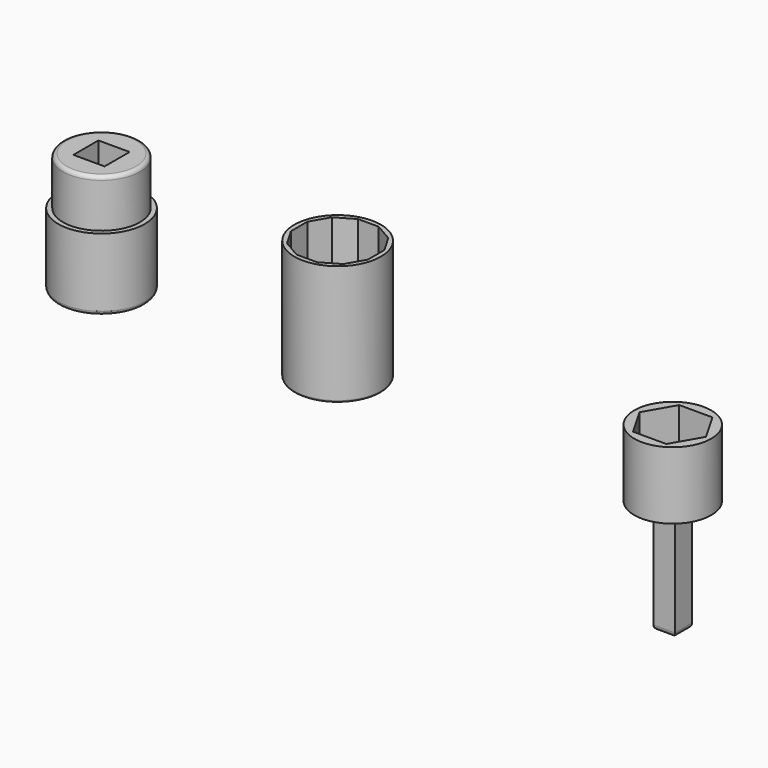
from build123d import *

# Parameters (mm, degrees)
F0_R      = 9
F0_W      = 10
F0_H      = 10
F1_DEPTH  = 12.5
F2_R      = 0.4
F3_R      = 9
F4_DEPTH  = 12.5
F6_DEPTH  = 10
F7_R      = 8
F8_DEPTH  = 14
F10_DEPTH = 23.5
F11_R     = 3.5
F12_DEPTH = 12
F13_R     = 1
F14_R     = 9
F15_DEPTH = 15
F16_R     = 8
F17_DEPTH = 10
F19_DEPTH = 14
F20_W     = 6.5
F20_H     = 6.5
F21_DEPTH = 25
F24_DEPTH = 10


# Not quite as in the source:
# - a fillet or chamfer that OpenCascade refuses, or shapes differently, is made with other operations: its cross-section is extruded or revolved along the edge and cut away or added
# - a feature names something its author has since deleted; it is built from what else it names


with BuildPart() as f1:
    # F0 (on Top) → F1 (new body)
    with BuildSketch(Plane.XY):
        Circle(F0_R)
        Rectangle(F0_W, F0_H, mode=Mode.SUBTRACT)
    extrude(amount=F1_DEPTH)

    # F2
    f2_edges = [f1.edges().sort_by_distance(p)[0] for p in [
        (-9, 0, 0),
    ]]
    fillet(f2_edges, radius=F2_R)

    # F3 (on face) → F4 (join)
    with BuildSketch(Plane.XY.offset(12.5)):
        Circle(F3_R)
    extrude(amount=F4_DEPTH)

    # F5 (on face) → F6 (cut)
    with BuildSketch(Plane.XY.offset(25)):
        Polygon((2.1435935394, 8), (-2.1435935394, 8), (-5.8564064606, 5.8564064606), (-8, 2.1435935394), (-8, -2.1435935394), (-5.8564064606, -5.8564064606), (-2.1435935394, -8), (2.1435935394, -8), (5.8564064606, -5.8564064606), (8, -2.1435935394), (8, 2.1435935394), (5.8564064606, 5.8564064606), align=None)
    extrude(amount=-F6_DEPTH, mode=Mode.SUBTRACT)

    # F11 (on face) → F12 (cut)
    with BuildSketch(Plane.XY.offset(15)):
        Circle(F11_R)
    extrude(amount=-F12_DEPTH, mode=Mode.SUBTRACT)


with BuildPart() as f8:
    # F7 (on Top) → F8 (new body)
    with BuildSketch(Plane.XY):
        with Locations((69.7127382428, 0)):
            Circle(F7_R)
    extrude(amount=F8_DEPTH)

    # F9 (on face) → F10 (join)
    with BuildSketch(Plane(origin=(0, 0, 0), x_dir=(1, 0, 0), z_dir=(0, 0, -1))):
        with BuildLine():
            Line((71.9627382428, -2.25), (71.9627382428, 0))
            ThreePointArc((71.9627382428, 0), (71.3037285004, -1.5909902577), (69.7127382428, -2.25))
            Line((69.7127382428, -2.25), (71.9627382428, -2.25))
        make_face()
        with BuildLine():
            ThreePointArc((69.7127382428, 2.25), (71.3037285004, 1.5909902577), (71.9627382428, 0))
            Line((71.9627382428, 0), (71.9627382428, 2.25))
            Line((71.9627382428, 2.25), (69.7127382428, 2.25))
        make_face()
        with BuildLine():
            Line((67.4627382428, -2.25), (69.7127382428, -2.25))
            ThreePointArc((69.7127382428, -2.25), (68.1217479851, -1.5909902577), (67.4627382428, 0))
            Line((67.4627382428, 0), (67.4627382428, -2.25))
        make_face()
        with BuildLine():
            ThreePointArc((69.7127382428, -2.25), (71.3037285004, -1.5909902577), (71.9627382428, 0))
            ThreePointArc((71.9627382428, 0), (71.3037285004, 1.5909902577), (69.7127382428, 2.25))
            ThreePointArc((69.7127382428, 2.25), (68.1217479851, 1.5909902577), (67.4627382428, 0))
            ThreePointArc((67.4627382428, 0), (68.1217479851, -1.5909902577), (69.7127382428, -2.25))
        make_face()
        with BuildLine():
            ThreePointArc((67.4627382428, 0), (68.1217479851, 1.5909902577), (69.7127382428, 2.25))
            Line((69.7127382428, 2.25), (67.4627382428, 2.25))
            Line((67.4627382428, 2.25), (67.4627382428, 0))
        make_face()
    extrude(amount=F10_DEPTH)

    # F13
    f13_edges = [f8.edges().sort_by_distance(p)[0] for p in [
        (69.712738, 2.25, -23.5),
        (71.962738, 0, -23.5),
        (69.712738, -2.25, -23.5),
        (67.462738, 0, -23.5),
    ]]
    fillet(f13_edges, radius=F13_R)

    # F23 (on face) → F24 (cut)
    with BuildSketch(Plane.XY.offset(14)):
        Polygon((73.1768398579, 6), (66.2486366276, 6), (62.7845350125, 0), (66.2486366276, -6), (73.1768398579, -6), (76.640941473, 0), align=None)
    extrude(amount=-F24_DEPTH, mode=Mode.SUBTRACT)


with BuildPart() as f15:
    # F14 (on Top) → F15 (new body)
    with BuildSketch(Plane.XY):
        with Locations((-49.1215325892, 0)):
            Circle(F14_R)
    extrude(amount=F15_DEPTH)

    # F16 (on face) → F17 (join)
    with BuildSketch(Plane.XY.offset(15)):
        with Locations((-49.1215325892, 0)):
            Circle(F16_R)
    extrude(amount=F17_DEPTH)

    # F18 (on face) → F19 (cut)
    with BuildSketch(Plane(origin=(0, 0, 0), x_dir=(1, 0, 0), z_dir=(0, 0, -1))):
        Polygon((-44.9404731584, 7.2629388451), (-53.2885253239, 7.2629388451), (-57.4625514066, 0.0333135977), (-53.2885253239, -7.1963116497), (-44.9404731584, -7.1963116497), (-40.7664470756, 0.0333135977), align=None)
    extrude(amount=-F19_DEPTH, mode=Mode.SUBTRACT)

    # F20 (on face) → F21 (cut)
    with BuildSketch(Plane.XY.offset(25)):
        with Locations((-49.1215325892, 0)):
            Rectangle(F20_W, F20_H)
    extrude(amount=-F21_DEPTH, mode=Mode.SUBTRACT)

    # F22: fillet of radius 0.8 on 2 edges, made by hand

    # F22_s1 → F22_t2 (revolve, cut)
    with BuildSketch(Plane.XZ):
        with BuildLine():
            ThreePointArc((-41.1211325892, 24.1990343146), (-41.3558471642, 24.7656854249), (-41.9224982746, 25.0004))
            Line((-41.9224982746, 25.0004), (-41.9224982746, 25.0805365685))
            ThreePointArc((-41.9224982746, 25.0805365685), (-41.5220154319, 25.0801365685), (-41.1215325892, 25.0801365685))
            Line((-41.1215325892, 25.0801365685), (-41.0413960207, 25))
            ThreePointArc((-41.0413960207, 25), (-41.0413960207, 24.5995171573), (-41.0409960207, 24.1990343146))
            Line((-41.0409960207, 24.1990343146), (-41.1211325892, 24.1990343146))
        make_face()
    revolve(axis=Axis((-49.1215325892, 0, 25), (0, 0, 1)), mode=Mode.SUBTRACT)

    # F22_s3 → F22_t4 (revolve, cut)
    with BuildSketch(Plane.XZ):
        with BuildLine():
            ThreePointArc((-40.1211325892, 0.8009656854), (-40.3558471642, 0.2343145751), (-40.9224982746, -0.0004))
            Line((-40.9224982746, -0.0004), (-40.9224982746, -0.0805365685))
            ThreePointArc((-40.9224982746, -0.0805365685), (-40.5220154319, -0.0801365685), (-40.1215325892, -0.0801365685))
            Line((-40.1215325892, -0.0801365685), (-40.0413960207, 0))
            ThreePointArc((-40.0413960207, 0), (-40.0413960207, 0.4004828427), (-40.0409960207, 0.8009656854))
            Line((-40.0409960207, 0.8009656854), (-40.1211325892, 0.8009656854))
        make_face()
    revolve(axis=Axis((-49.1215325892, 0, 0), (0, 0, 1)), mode=Mode.SUBTRACT)


solid = Compound([f1.part, f8.part, f15.part])
